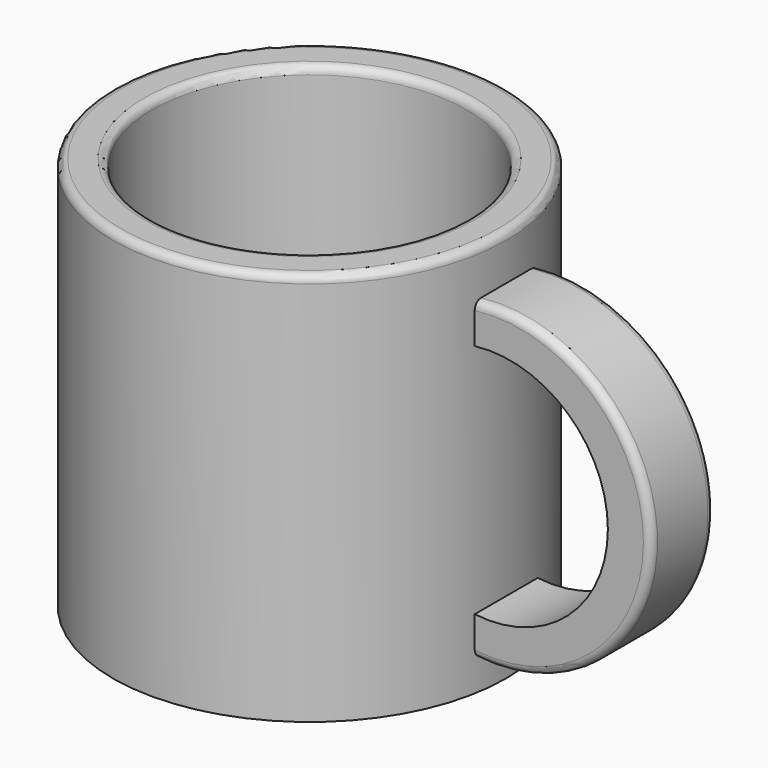
from build123d import *

# Parameters (mm, degrees)
F3_DEPTH = 10
F4_DEPTH = 10
F6_R     = 2


# Not quite as in the source:
# - a fillet or chamfer that OpenCascade refuses, or shapes differently, is made with other operations: its cross-section is extruded or revolved along the edge and cut away or added


with BuildPart() as f1:
    # F0 (on Front) → F1 (revolve)
    with BuildSketch(Plane.XZ):
        Polygon((-50, 0), (0, 0), (0, 100), (-10, 100), (-10, 10), (-50, 10), align=None)
    revolve(axis=Axis((-50, 0, 5), (0, 0, -1)))

    # F2 (on Front) → F3 (join)
    with BuildSketch(Plane.XZ):
        with BuildLine():
            Line((0, 18.4238510507), (0, 8.4238510507))
            ThreePointArc((0, 8.4238510507), (44.875886677, 48.4238510507), (0, 88.4238510507))
            Line((0, 88.4238510507), (0, 78.4238510507))
            ThreePointArc((0, 78.4238510507), (33.8383705003, 48.4238510507), (0, 18.4238510507))
        make_face()
    extrude(amount=F3_DEPTH)

    # F2 (on Front) → F4 (join)
    with BuildSketch(Plane.XZ):
        with BuildLine():
            Line((0, 18.4238510507), (0, 8.4238510507))
            ThreePointArc((0, 8.4238510507), (44.875886677, 48.4238510507), (0, 88.4238510507))
            Line((0, 88.4238510507), (0, 78.4238510507))
            ThreePointArc((0, 78.4238510507), (33.8383705003, 48.4238510507), (0, 18.4238510507))
        make_face()
    extrude(amount=-F4_DEPTH)

    # F5: fillet of radius 2 on 2 edges, made by hand

    # F5_s1 → F5_t2 (revolve, cut)
    with BuildSketch(Plane.XZ):
        with BuildLine():
            ThreePointArc((0, 98), (-0.5857864376, 99.4142135624), (-2, 100))
            Line((-2, 100), (0, 100))
            Line((0, 100), (0, 98))
        make_face()
    revolve(axis=Axis((-50, 0, 100), (0, 0, -1)), mode=Mode.SUBTRACT)

    # F5_s3 → F5_t4 (revolve, cut)
    with BuildSketch(Plane.XZ):
        with BuildLine():
            ThreePointArc((-8, 100), (-9.4142135624, 99.4142135624), (-10, 98))
            Line((-10, 98), (-10, 100))
            Line((-10, 100), (-8, 100))
        make_face()
    revolve(axis=Axis((-50, 0, 100), (0, 0, -1)), mode=Mode.SUBTRACT)

    # F6
    f6_edges = [f1.edges().sort_by_distance(p)[0] for p in [
        (44.875887, -10, 48.423851),
        (44.875887, 10, 48.423851),
    ]]
    fillet(f6_edges, radius=F6_R)


solid = f1.part
